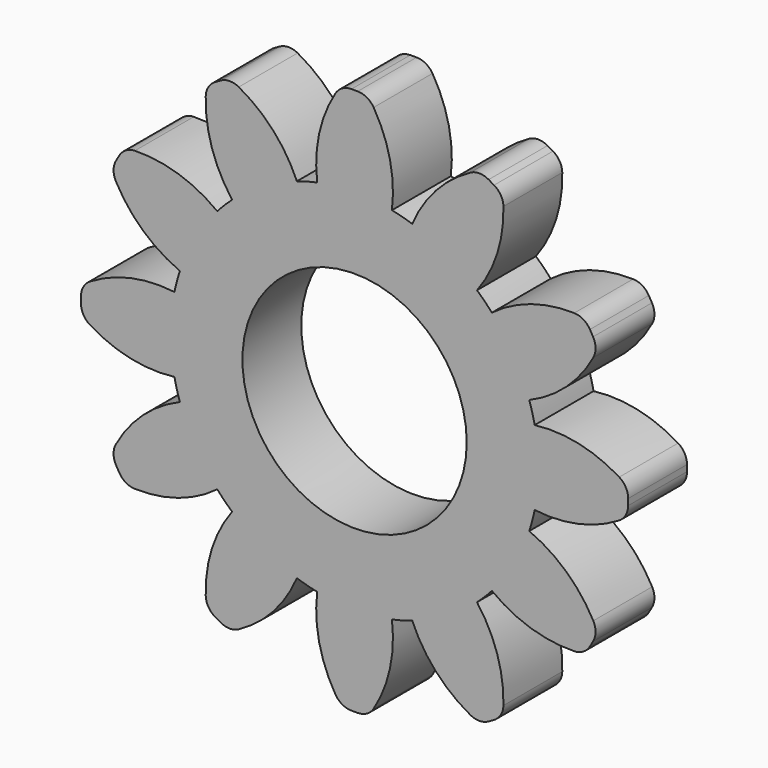
from build123d import *

# Parameters (mm, degrees)
F0_R     = 12.5
F1_DEPTH = 5
F3_DEPTH = 5
F4_R     = 1.27
F5_COUNT = 12
F6_R     = 7.62
F7_DEPTH = 25.4


with BuildPart() as f1:
    # F0 (on Front) → F1 (new body)
    with BuildSketch(Plane.XZ):
        Circle(F0_R)
    extrude(amount=F1_DEPTH)

    # F2 (on face) → F3 (join, through all)
    with BuildSketch(Plane.XZ.offset(5)):
        with BuildLine():
            ThreePointArc((-2.54, 12.2392156611), (0, 12.5), (2.54, 12.2392156611))
            ThreePointArc((2.54, 12.2392156611), (2.3217431159, 15.5720988713), (0.889, 18.5892156611))
            Line((0.889, 18.5892156611), (-0.889, 18.5892156611))
            ThreePointArc((-0.889, 18.5892156611), (-2.3217431159, 15.5720988713), (-2.54, 12.2392156611))
        make_face()
    extrude(amount=-F3_DEPTH)

    # F4
    f4_edges = [f1.edges().sort_by_distance(p)[0] for p in [
        (-0.889, -2.5, 18.589216),
        (0.889, -2.5, 18.589216),
    ]]
    fillet(f4_edges, radius=F4_R)

    # F5: F1 ×12 about axis
    f5_axis = Axis((0, 0, 0), (0, 1, 0))


with BuildPart() as f1_1:
    add(f1.part)
    for i in range(1, F5_COUNT):
        add(f1.part.rotate(f5_axis, i * 360 / F5_COUNT))

    # F6 (on face) → F7 (cut)
    with BuildSketch(Plane.XZ.offset(5)):
        Circle(F6_R)
    extrude(amount=-F7_DEPTH, mode=Mode.SUBTRACT)


solid = f1_1.part
